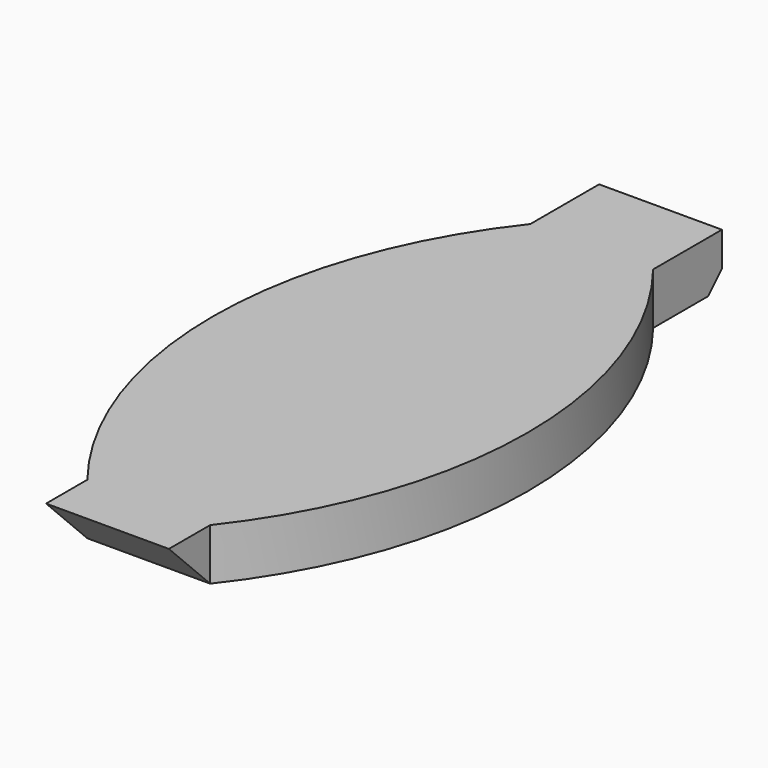
from build123d import *

# Parameters (mm, degrees)
F1_DEPTH    = 3.81
F2_W        = 9.0688861602
F2_H        = 3.81
F3_DEPTH    = 6.35
F4_SIZE     = 1.27
F5_W        = 9.0688861602
F5_H        = 3.81
F6_DEPTH    = 5.08
F7_T1_DEPTH = 35.1971853179
F8_R        = 0.9525
F9_DEPTH    = 8.89


# Not quite as in the source:
# - a fillet or chamfer that OpenCascade refuses, or shapes differently, is made with other operations: its cross-section is extruded or revolved along the edge and cut away or added


with BuildPart() as f1:
    # F0 (on Top) → F1 (new body)
    with BuildSketch(Plane.XY):
        with BuildLine():
            Line((4.5344430801, -2.4189800566), (-4.5344430801, -2.4189800566))
            ThreePointArc((-4.5344430801, -2.4189800566), (-11.6244136954, -22.8629027748), (-4.5344430801, -43.306825493))
            Line((-4.5344430801, -43.306825493), (4.5344430801, -43.306825493))
            ThreePointArc((4.5344430801, -43.306825493), (11.6244136954, -22.8629027748), (4.5344430801, -2.4189800566))
        make_face()
    extrude(amount=F1_DEPTH)

    # F2 (on face) → F3 (join)
    with BuildSketch(Plane(origin=(0, -2.4189800566, 0), x_dir=(-1, 0, 0), z_dir=(0, 1, 0))):
        with Locations((0, 1.905)):
            Rectangle(F2_W, F2_H)
    extrude(amount=F3_DEPTH)

    # F4
    f4_edges = [f1.edges().sort_by_distance(p)[0] for p in [
        (0, 3.93102, 0),
    ]]
    chamfer(f4_edges, length=F4_SIZE)

    # F5 (on face) → F6 (join)
    with BuildSketch(Plane.XZ.offset(43.306825493)):
        with Locations((0, 1.905)):
            Rectangle(F5_W, F5_H)
    extrude(amount=F6_DEPTH)

    # F7: chamfer of 5.08 on 1 edges, made by hand

    # F7_s2 → F7_t1 (cut)
    with BuildSketch(Plane.YZ.offset(-17.598592659)):
        Polygon((-43.306825493, 0), (-48.386825493, 5.08), (-48.386825493, 0), align=None)
    extrude(amount=F7_T1_DEPTH, mode=Mode.SUBTRACT)

    # F8 (on face) → F9 (cut)
    with BuildSketch(Plane(origin=(0, 3.9310199434, 0), x_dir=(-1, 0, 0), z_dir=(0, 1, 0))):
        with Locations((0, 2.4971892126)):
            Circle(F8_R)
    extrude(amount=-F9_DEPTH, mode=Mode.SUBTRACT)


solid = f1.part
